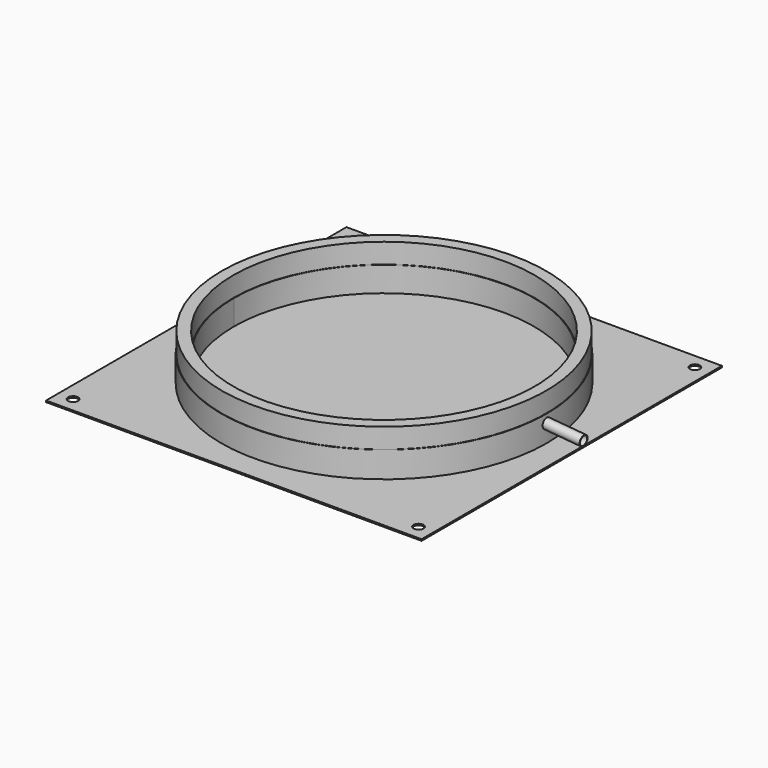
from build123d import *
from build123d import SkipClean  # not in build123d's __all__

# Parameters (mm, degrees)
F0_W     = 10
F0_H     = 3
F2_W     = 750
F2_H     = 750
F2_R     = 10
F3_DEPTH = 3
F6_R     = 9
F7_DEPTH = 120
F8_R     = 300
F9_DEPTH = 200


with BuildPart() as f1:
    # F0 (on Front) → F1 (revolve)
    with BuildSketch(Plane.XZ):
        Polygon((-325, 5), (-300, 5), (-300, 55), (-301, 55), (-301, 95), (-324, 95), (-324, 55), (-325, 55), align=None)
        Polygon((-10, 5), (-300, 5), (-325, 5), (-325, 2), (-10, 2), align=None)
        with Locations((-5, 3.5)):
            Rectangle(F0_W, F0_H)
    revolve(axis=Axis((0, 0, 187.9212413023), (0, 0, -1)))

    # F2 (on Top) → F3 (join)
    with BuildSketch(Plane.XY):
        Rectangle(F2_W, F2_H)
        with Locations((-345, -345)):
            Circle(F2_R, mode=Mode.SUBTRACT)
        with Locations((345, -345)):
            Circle(F2_R, mode=Mode.SUBTRACT)
        with Locations((-345, 345)):
            Circle(F2_R, mode=Mode.SUBTRACT)
        with Locations((345, 345)):
            Circle(F2_R, mode=Mode.SUBTRACT)
    extrude(amount=F3_DEPTH)

    # F4 (on Front) → F5 (revolve)
    with BuildSketch(Plane.XZ):
        Polygon((399.6194698092, 41.5098406888), (300, 50.2254149636), (299.9128442573, 49.2292202655), (399.5323140664, 40.5136459907), align=None)
    revolve(axis=Axis((412.7442754949, 0, 30.3233706049), (0.9961946981, 0, -0.0871557427)))

    # F6 (on face) → F7 (cut)
    with BuildSketch(Plane(origin=(392.9798568705, 0, -34.3812824702), x_dir=(0, 1, 0), z_dir=(0.9961946981, 0, -0.0871557427))):
        with Locations((0, 66.1810149205)):
            Circle(F6_R)
    extrude(amount=-F7_DEPTH, mode=Mode.SUBTRACT)

    # F8 (on face) → F9 (cut)
    with BuildSketch(Plane.XY.offset(5)):
        Circle(F8_R)
    with SkipClean():  # cleaning this boolean's faces spoils the solid; the shape is the same uncleaned
        extrude(amount=F9_DEPTH, mode=Mode.SUBTRACT)


solid = f1.part
